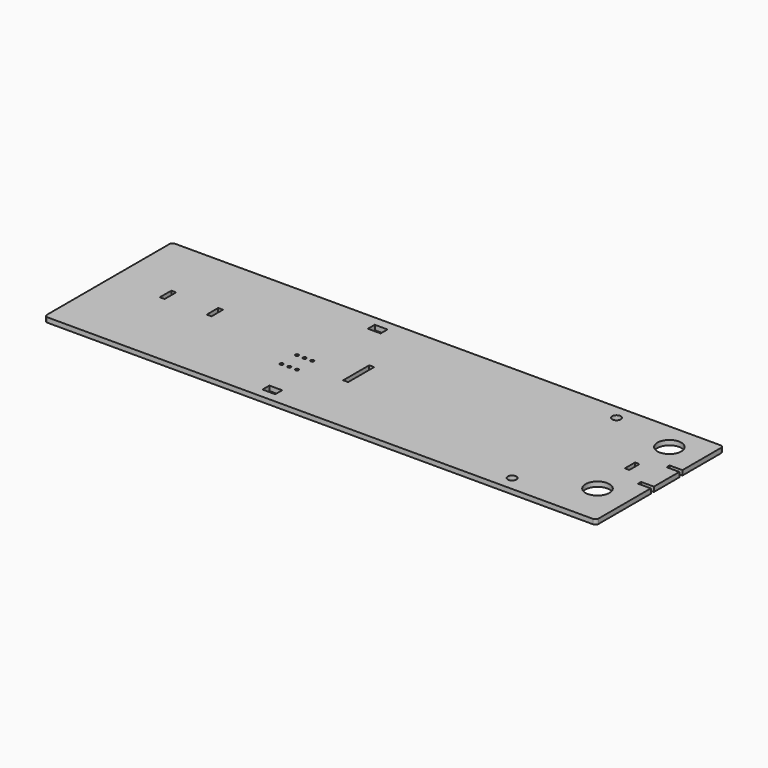
from build123d import *

# Parameters (mm, degrees)
F0_W      = 173
F0_H      = 50
F1_DEPTH  = 1.5
F2_W      = 1.5
F2_H      = 4.5
F4_DEPTH  = 1.501
F3_W      = 1.5
F3_H      = 4.5
F5_DEPTH  = 1.501
F6_W      = 4
F6_H      = 2.7
F7_DEPTH  = 1.501
F8_R      = 1.35
F9_DEPTH  = 1.501
F10_R     = 3.75
F11_DEPTH = 1.501
F12_W     = 4
F12_H     = 1.2
F13_DEPTH = 1.501
F14_W     = 1.4
F14_H     = 4
F15_DEPTH = 1.501
F16_R     = 1
F17_R     = 0.5
F18_DEPTH = 1.501
F19_W     = 1.5543582849
F19_H     = 10.2004739456
F20_DEPTH = 1.501


# Not quite as in the source:
# - a pattern or mirror of a feature is missing from the dataset's text; its kind, count and spacing are read off the source's solid


with BuildPart() as f1:
    # F0 (on Top) → F1 (new body)
    with BuildSketch(Plane.XY):
        Rectangle(F0_W, F0_H)
    extrude(amount=F1_DEPTH)

    # F2 (on face) → F4 (cut, through all)
    with BuildSketch(Plane.XY.offset(1.5)):
        with Locations((-69.95, 2.75)):
            Rectangle(F2_W, F2_H)
    extrude(amount=-F4_DEPTH, mode=Mode.SUBTRACT)

    # F3 (on face) → F5 (cut, through all)
    with BuildSketch(Plane.XY.offset(1.5)):
        with Locations((-55.25, 2.75)):
            Rectangle(F3_W, F3_H)
    extrude(amount=-F5_DEPTH, mode=Mode.SUBTRACT)

    # F6 (on face) → F7 (cut, through all)
    with BuildSketch(Plane.XY.offset(1.5)):
        with Locations((-18.5, 20.65)):
            Rectangle(F6_W, F6_H)
    f7 = extrude(amount=-F7_DEPTH, mode=Mode.SUBTRACT)

    # F7_copies: F7 across plane
    add(f7.mirror(Plane(origin=(0, 0, 0), x_dir=(0, 0, -1), z_dir=(0, -1, 0))), mode=Mode.SUBTRACT)

    # F8 (on face) → F9 (cut, through all)
    with BuildSketch(Plane.XY.offset(1.5)):
        with Locations((56.55, 20.45)):
            Circle(F8_R)
    f9 = extrude(amount=-F9_DEPTH, mode=Mode.SUBTRACT)

    # F9_copies: F9 across plane
    add(f9.mirror(Plane(origin=(0, 0, 0), x_dir=(0, 0, -1), z_dir=(0, -1, 0))), mode=Mode.SUBTRACT)

    # F10 (on face) → F11 (cut, through all)
    with BuildSketch(Plane.XY.offset(1.5)):
        with Locations((76.35, 16.45)):
            Circle(F10_R)
        with Locations((76.35, -11.75)):
            Circle(F10_R)
    extrude(amount=-F11_DEPTH, mode=Mode.SUBTRACT)

    # F12 (on face) → F13 (cut, through all)
    with BuildSketch(Plane.XY.offset(1.5)):
        with Locations((84.5, 8.2552298188)):
            Rectangle(F12_W, F12_H)
        with Locations((84.5, -2.9447701812)):
            Rectangle(F12_W, F12_H)
    extrude(amount=-F13_DEPTH, mode=Mode.SUBTRACT)

    # F14 (on face) → F15 (cut, through all)
    with BuildSketch(Plane.XY.offset(1.5)):
        with Locations((75.6, 2.8)):
            Rectangle(F14_W, F14_H)
    extrude(amount=-F15_DEPTH, mode=Mode.SUBTRACT)

    # F16
    f16_edges = [f1.edges().sort_by_distance(p)[0] for p in [
        (-86.5, -25, 0.75),
        (-86.5, 25, 0.75),
        (86.5, 25, 0.75),
        (86.5, -25, 0.75),
    ]]
    fillet(f16_edges, radius=F16_R)

    # F17 (on face) → F18 (cut, through all)
    with BuildSketch(Plane.XY.offset(1.5)):
        with Locations((-25.3, -2.5)):
            Circle(F17_R)
        with Locations((-22.9, -2.5)):
            Circle(F17_R)
        with Locations((-20.5, -2.5)):
            Circle(F17_R)
        with Locations((-20.5, -8.5)):
            Circle(F17_R)
        with Locations((-22.9, -8.5)):
            Circle(F17_R)
        with Locations((-25.3, -8.5)):
            Circle(F17_R)
    extrude(amount=-F18_DEPTH, mode=Mode.SUBTRACT)

    # F19 (on face) → F20 (cut, through all)
    with BuildSketch(Plane.XY.offset(1.5)):
        with Locations((-7.3602499906, -0.7336952258)):
            Rectangle(F19_W, F19_H)
    extrude(amount=-F20_DEPTH, mode=Mode.SUBTRACT)


solid = f1.part
